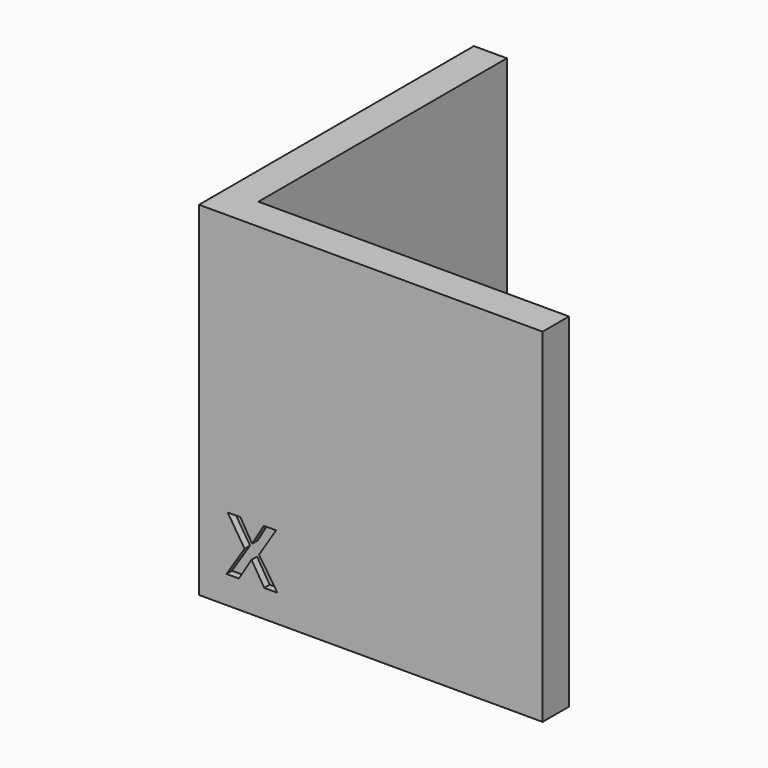
from build123d import *

# Parameters (mm, degrees)
F1_DEPTH     = 25
F2_TEXT_SIZE = 5.5555555556
F3_DEPTH     = 0.5
F4_TEXT_SIZE = 5.5555555556
F5_DEPTH     = 0.5


# Not quite as in the source:
# - Text() gives the source's letters only with a copy of the font that has no kerning and outlines rounded to 1/6400 em; it was checked with that copy


with BuildPart() as f1:
    # F0 (on Top) → F1 (new body)
    with BuildSketch(Plane.XY):
        Polygon((0, 25), (0, 0), (25, 0), (25, 2.4), (2.4, 2.4), (2.4, 25), align=None)
    extrude(amount=F1_DEPTH)

    # F2 (on face) → F3 (cut)
    with BuildSketch(Plane.XZ):
        with Locations((2, 2)):
            Text('X', F2_TEXT_SIZE, font='Open Sans', font_style=FontStyle.BOLD, text_align=(TextAlign.LEFT, TextAlign.BOTTOM))
    extrude(amount=-F3_DEPTH, mode=Mode.SUBTRACT)

    # F4 (on face) → F5 (cut)
    with BuildSketch(Plane(origin=(0, 0, 0), x_dir=(0, -1, 0), z_dir=(-1, 0, 0))):
        with Locations((-5.8272569444, 2)):
            Text('Y', F4_TEXT_SIZE, font='Open Sans', font_style=FontStyle.BOLD, text_align=(TextAlign.LEFT, TextAlign.BOTTOM))
    extrude(amount=-F5_DEPTH, mode=Mode.SUBTRACT)


solid = f1.part
